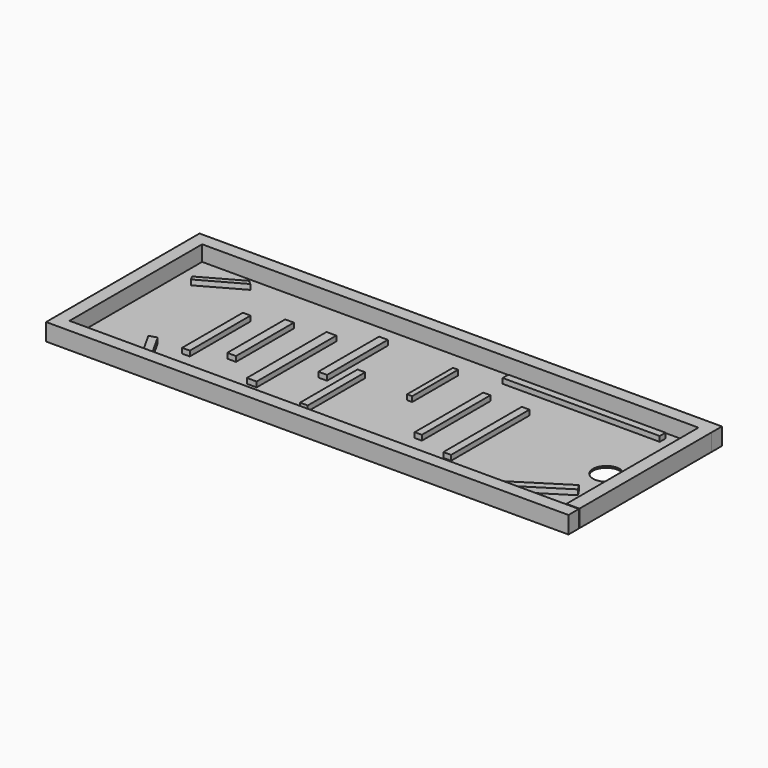
from build123d import *

# Parameters (mm, degrees)
F2_DEPTH = 25.4
F0_W     = 48.0314
F0_H     = 608.6317263126
F3_DEPTH = 63.5
F0_W_2   = 1828.8
F0_H_2   = 609.6
F0_W_3   = 28.3958315849
F0_H_3   = 280.1721617579
F0_H_4   = 265.0277093053
F0_W_4   = 35.9680652618
F0_H_5   = 367.2526776791
F0_W_5   = 26.5027880669
F0_H_6   = 316.140204668
F0_H_7   = 361.5735173225
F0_W_6   = 32.1819484234
F0_H_8   = 266.9207602739
F0_W_7   = 32.1819335222
F0_H_9   = 280.1721505821
F0_W_8   = 18.93055439
F0_H_10  = 211.7604613304
F0_R     = 49.3032271109
F0_W_9   = 579.2748481035
F0_H_11  = 26.5027880669
F4_DEPTH = 6.35
F5_DEPTH = 25.4
F7_DEPTH = 25.4
F8_DEPTH = 25.4


# Not quite as in the source:
# - the program builds the solid bodies; features that only make, move or delete a surface that nothing else refers to are left out


with BuildPart() as f2:
    # F0 (on Top) → F2 (new body)
    with BuildSketch(Plane.XY):
        Polygon((-724.242739406, -180.6030766776), (-664.2644405365, -288.006067276), (-639.6492631828, -274.2599280315), (-696.7837155241, -171.9494063374), align=None)
    extrude(amount=F2_DEPTH)


with BuildPart() as f3:
    # F0 (on Top) → F3 (new body)
    with BuildSketch(Plane.XY):
        Polygon((-914.4, -306.5295712601), (-914.4, -304.8), (-914.4, 304.8), (-962.4407291412, 304.8), (-962.4407291412, -306.5295712601), align=None)
        Polygon((964.4395112991, -306.5295712601), (-914.4, -306.5295712601), (-962.4407291412, -306.5295712601), (-962.4407291412, -354.5609712601), (964.4395112991, -354.5609712601), align=None)
        Polygon((-962.4407291412, 304.8), (-914.4, 304.8), (914.4, 304.8), (916.3329601288, 304.8), (964.3643601288, 304.8), (964.4395112991, 304.8), (964.4395112991, 352.8314), (-962.4407291412, 352.8314), align=None)
        with Locations((940.3486601288, 0.4841368437)):
            Rectangle(F0_W, F0_H)
    extrude(amount=F3_DEPTH)


with BuildPart() as f4:
    # F0 (on Top) → F4 (new body)
    with BuildSketch(Plane.XY):
        Rectangle(F0_W_2, F0_H_2)
        Polygon((-639.6492631828, -274.2599280315), (-664.2644405365, -288.006067276), (-724.242739406, -180.6030766776), (-696.7837155241, -171.9494063374), align=None, mode=Mode.SUBTRACT)
        with Locations((-587.59573102, -38.1228066981)):
            Rectangle(F0_W_3, F0_H_3, mode=Mode.SUBTRACT)
        with Locations((-108.6528003216, -100.5936227739)):
            Rectangle(F0_W_3, F0_H_4, mode=Mode.SUBTRACT)
        with Locations((-320.6749558449, -24.8714238405)):
            Rectangle(F0_W_4, F0_H_5, mode=Mode.SUBTRACT)
        Polygon((652.9883329754, -274.2599280315), (634.3713402748, -253.9310753345), (825.5698084831, -132.7755451202), (840.0946035245, -155.6974749573), align=None, mode=Mode.SUBTRACT)
        with Locations((263.332515955, -12.5665664673)):
            Rectangle(F0_W_5, F0_H_6, mode=Mode.SUBTRACT)
        with Locations((406.2581658363, -35.2832227945)):
            Rectangle(F0_W_3, F0_H_7, mode=Mode.SUBTRACT)
        with Locations((-464.5471423864, 12.0431557298)):
            Rectangle(F0_W_6, F0_H_8, mode=Mode.SUBTRACT)
        with Locations((-186.2680539489, 90.6049404293)):
            Rectangle(F0_W_7, F0_H_9, mode=Mode.SUBTRACT)
        Polygon((-857.3560714722, 187.1507465839), (-711.5908265114, 268.5521245003), (-696.7837155241, 255.1123515359), (-848.1149500553, 170.6026934488), align=None, mode=Mode.SUBTRACT)
        with Locations((94.8506072164, 105.8802306652)):
            Rectangle(F0_W_8, F0_H_10, mode=Mode.SUBTRACT)
        with Locations((820.462346077, 0)):
            Circle(F0_R, mode=Mode.SUBTRACT)
        with Locations((526.467166841, 264.7660076618)):
            Rectangle(F0_W_9, F0_H_11, mode=Mode.SUBTRACT)
    extrude(amount=F4_DEPTH)

    # F0 (on Top) → F5 (join)
    with BuildSketch(Plane.XY):
        with Locations((-587.59573102, -38.1228066981)):
            Rectangle(F0_W_3, F0_H_3)
        Polygon((-696.7837155241, 255.1123515359), (-711.5908265114, 268.5521245003), (-857.3560714722, 187.1507465839), (-848.1149500553, 170.6026934488), align=None)
        with Locations((-464.5471423864, 12.0431557298)):
            Rectangle(F0_W_6, F0_H_8)
        with Locations((-320.6749558449, -24.8714238405)):
            Rectangle(F0_W_4, F0_H_5)
        with Locations((-186.2680539489, 90.6049404293)):
            Rectangle(F0_W_7, F0_H_9)
        with Locations((-108.6528003216, -100.5936227739)):
            Rectangle(F0_W_3, F0_H_4)
        with Locations((94.8506072164, 105.8802306652)):
            Rectangle(F0_W_8, F0_H_10)
        with Locations((263.332515955, -12.5665664673)):
            Rectangle(F0_W_5, F0_H_6)
        with Locations((406.2581658363, -35.2832227945)):
            Rectangle(F0_W_3, F0_H_7)
    extrude(amount=F5_DEPTH)

    # F0 (on Top) → F7 (join)
    with BuildSketch(Plane.XY):
        with Locations((526.467166841, 264.7660076618)):
            Rectangle(F0_W_9, F0_H_11)
    extrude(amount=F7_DEPTH)

    # F0 (on Top) → F8 (join)
    with BuildSketch(Plane.XY):
        Polygon((825.5698084831, -132.7755451202), (634.3713402748, -253.9310753345), (652.9883329754, -274.2599280315), (840.0946035245, -155.6974749573), align=None)
    extrude(amount=F8_DEPTH)


solid = Compound([f2.part, f3.part, f4.part])
